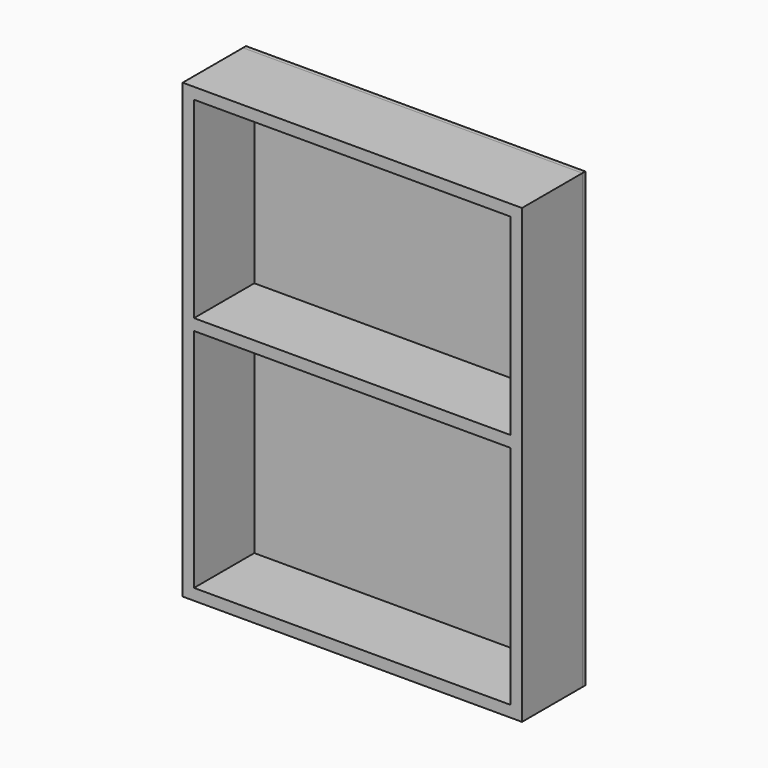
from build123d import *

# Parameters (mm, degrees)
F0_W     = 450
F0_H     = 100
F1_DEPTH = 15
F2_W     = 15
F2_H     = 100
F3_DEPTH = 570
F4_W     = 435
F4_H     = 100
F4_W_2   = 15
F5_DEPTH = 15
F6_W     = 100
F6_H     = 15
F7_DEPTH = 420
F8_W     = 450
F8_H     = 600
F8_W_2   = 420
F8_H_2   = 300
F8_H_3   = 255
F9_DEPTH = 5


with BuildPart() as f1:
    # F0 (on Top) → F1 (new body)
    with BuildSketch(Plane.XY):
        with Locations((225, 50)):
            Rectangle(F0_W, F0_H)
    extrude(amount=F1_DEPTH)

    # F2 (on face) → F3 (join)
    with BuildSketch(Plane.XY.offset(15)):
        with Locations((7.5, 50)):
            Rectangle(F2_W, F2_H)
        with Locations((442.5, 50)):
            Rectangle(F2_W, F2_H)
    extrude(amount=F3_DEPTH)

    # F4 (on face) → F5 (join)
    with BuildSketch(Plane.XY.offset(585)):
        with Locations((217.5, 50)):
            Rectangle(F4_W, F4_H)
        with Locations((442.5, 50)):
            Rectangle(F4_W_2, F4_H)
    extrude(amount=F5_DEPTH)

    # F6 (on face) → F7 (join, through all)
    with BuildSketch(Plane.YZ.offset(15)):
        with Locations((50, 322.5)):
            Rectangle(F6_W, F6_H)
    extrude(amount=F7_DEPTH)


with BuildPart() as f9:
    # F8 (on face) → F9 (new body)
    with BuildSketch(Plane(origin=(0, 100, 0), x_dir=(-1, 0, 0), z_dir=(0, 1, 0))):
        with Locations((-225, 300)):
            Rectangle(F8_W, F8_H)
        with Locations((-225, 165)):
            Rectangle(F8_W_2, F8_H_2, mode=Mode.SUBTRACT)
        with Locations((-225, 457.5)):
            Rectangle(F8_W_2, F8_H_3, mode=Mode.SUBTRACT)
        with Locations((-225, 457.5)):
            Rectangle(F8_W_2, F8_H_3)
        with Locations((-225, 165)):
            Rectangle(F8_W_2, F8_H_2)
    extrude(amount=F9_DEPTH)


solid = Compound([f1.part, f9.part])
